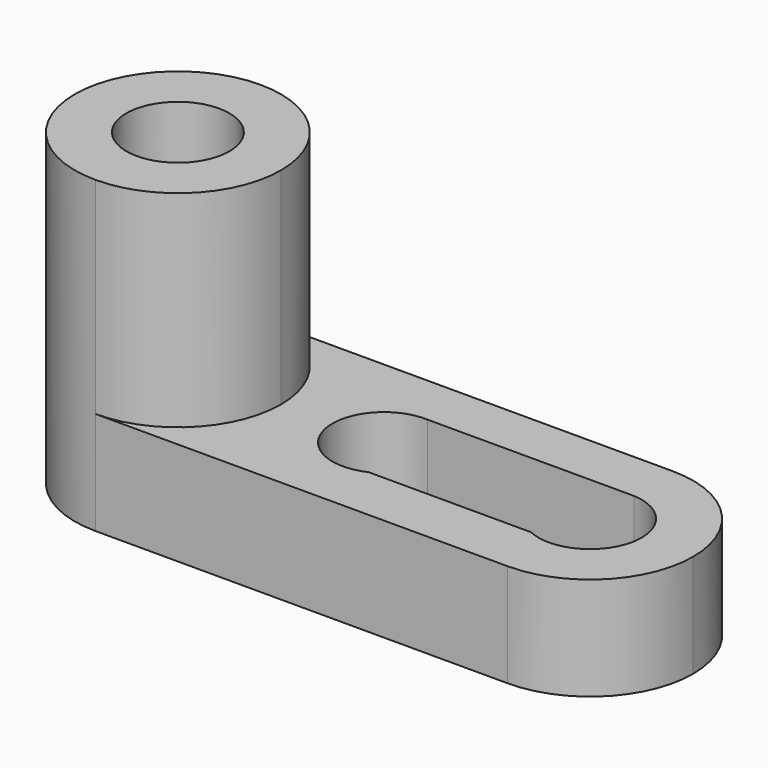
from build123d import *

# Parameters (mm, degrees)
F1_DEPTH = 25.4
F2_R     = 12.69999
F3_R     = 6.35
F4_DEPTH = 50.8
F5_R     = 12.69999
F6_R     = 6.35
F8_DEPTH = 25.4


# Not quite as in the source:
# - a fillet or chamfer is up to 0.001 mm smaller than in the source, because OpenCascade refuses the exact size


with BuildPart() as f1:
    # F0 (on Front) → F1 (new body)
    with BuildSketch(Plane.XZ):
        Polygon((0, 38.1), (0, 0), (76.2, 0), (76.2, 12.7), (25.4, 12.7), (25.4, 38.1), align=None)
    extrude(amount=F1_DEPTH)

    # F2 (radius 12.7 in the source; OpenCascade refuses exactly that, so slightly less here)
    f2_edges = [f1.edges().sort_by_distance(p)[0] for p in [
        (25.4, 0, 25.4),
        (25.4, -25.4, 25.4),
        (0, -25.4, 19.05),
        (0, 0, 19.05),
    ]]
    fillet(f2_edges, radius=F2_R)

    # F3 (on face) → F4 (cut)
    with BuildSketch(Plane.XY.offset(38.1)):
        with Locations((12.7, -12.7)):
            Circle(F3_R)
    extrude(amount=-F4_DEPTH, mode=Mode.SUBTRACT)

    # F5 (radius 12.7 in the source; OpenCascade refuses exactly that, so slightly less here)
    f5_edges = [f1.edges().sort_by_distance(p)[0] for p in [
        (76.2, 0, 6.35),
        (76.2, -25.4, 6.35),
    ]]
    fillet(f5_edges, radius=F5_R)

    # F6 (on face) + F7 (on face) → F8 (cut)
    with BuildSketch(Plane.XY.offset(12.7)):
        with Locations((38.1, -12.7)):
            Circle(F6_R)
    with BuildSketch(Plane.XY.offset(12.7)):
        with BuildLine():
            Line((40.7903380557, -18.4519197792), (60.8096619443, -18.4519197792))
            ThreePointArc((60.8096619443, -18.4519197792), (57.2698982045, -11.4718584702), (63.1938608334, -6.3573839143))
            Line((63.1938608334, -6.3573839143), (38.4061391666, -6.3573839143))
            ThreePointArc((38.4061391666, -6.3573839143), (42.6970905858, -8.3194454522), (44.45, -12.7))
            ThreePointArc((44.45, -12.7), (43.4575249254, -16.108728014), (40.7903380557, -18.4519197792))
        make_face()
        with BuildLine():
            ThreePointArc((63.1938608334, -6.3573839143), (57.2698982045, -11.4718584702), (60.8096619443, -18.4519197792))
            ThreePointArc((60.8096619443, -18.4519197792), (66.908728014, -18.0575249254), (69.85, -12.7))
            ThreePointArc((69.85, -12.7), (68.0970905858, -8.3194454522), (63.8061391666, -6.3573839143))
            Line((63.8061391666, -6.3573839143), (63.1938608334, -6.3573839143))
        make_face()
    extrude(amount=-F8_DEPTH, mode=Mode.SUBTRACT)


solid = f1.part
